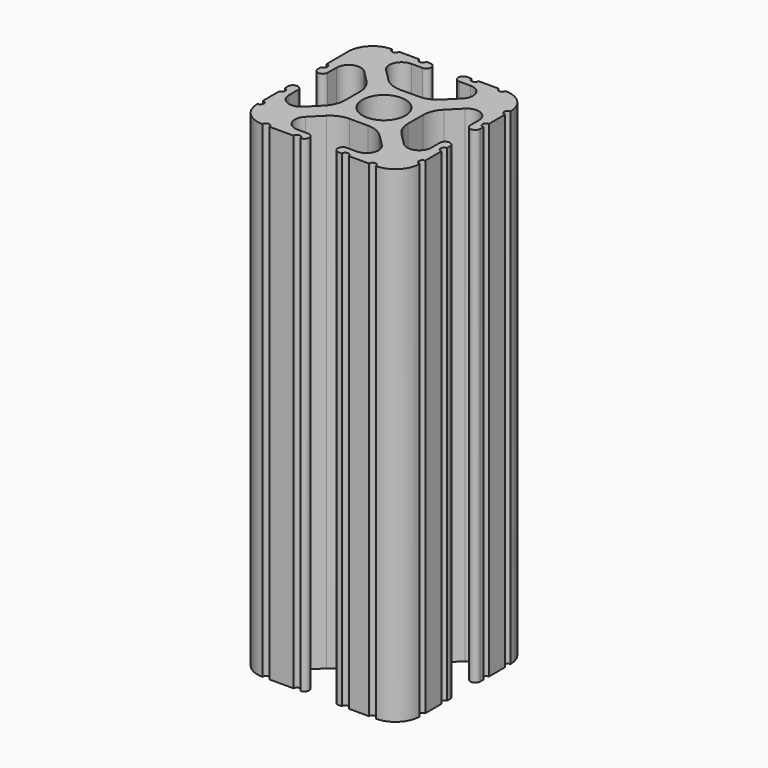
from build123d import *

# Parameters (mm, degrees)
F0_R     = 3.3625011168
F1_DEPTH = 76.2


# Not quite as in the source:
# - ends of sketch curves that miss each other by under 0.0002 mm in the source are joined


with BuildPart() as f1:
    # F0 (on Top) → F1 (new body)
    with BuildSketch(Plane.XY):
        with BuildLine():
            ThreePointArc((-8.5485764575, 18.7552378401), (-9.7846294165, 17.9293336576), (-11.2426532939, 17.6393146764))
            Line((-11.2426532939, 17.6393146764), (-14.1573467061, 17.6393146764))
            ThreePointArc((-14.1573467061, 17.6393146764), (-15.6153705835, 17.9293336576), (-16.8514235425, 18.7552378401))
            Line((-16.8514235425, 18.7552378401), (-18.696905198, 20.6007194956))
            ThreePointArc((-18.696905198, 20.6007194956), (-19.1098572893, 22.6767698525), (-17.3498667798, 23.8527579138))
            Line((-17.3498667798, 23.8527579138), (-15.6153705835, 23.8527579138))
            Line((-15.6153705835, 23.8527579138), (-15.5830195394, 23.8527579138))
            ThreePointArc((-15.5830195394, 23.8527579138), (-14.8254049311, 24.6263789569), (-15.5830195394, 25.4))
            Line((-15.5830195394, 25.4), (-15.6153705835, 25.4))
            Line((-15.6153705835, 25.4), (-16.2533409894, 25.4))
            ThreePointArc((-16.2533409894, 25.4), (-16.8016038846, 24.8587722652), (-17.3498667798, 25.4))
            Line((-17.3498667798, 25.4), (-20.4874817282, 25.4))
            ThreePointArc((-20.4874817282, 25.4), (-21.0387408641, 24.8487408595), (-21.5900000046, 25.4))
            ThreePointArc((-21.5900000046, 25.4), (-24.2840768363, 24.2840768363), (-25.4, 21.59))
            Line((-25.4, 21.59), (-25.4, 20.5047242343))
            Line((-25.4, 20.5047242343), (-25.4, 17.3498667798))
            ThreePointArc((-25.4, 17.3498667798), (-24.8441605755, 16.8026749055), (-25.4, 16.2554830313))
            Line((-25.4, 16.2554830313), (-25.4, 15.6153705835))
            ThreePointArc((-25.4, 15.6153705835), (-24.6263789569, 14.8595541131), (-23.8527579138, 15.6153705835))
            Line((-23.8527579138, 15.6153705835), (-23.8527579138, 17.3498667798))
            ThreePointArc((-23.8527579138, 17.3498667798), (-22.6767698525, 19.1098572893), (-20.6007194956, 18.696905198))
            Line((-20.6007194956, 18.696905198), (-18.7552378401, 16.8514235425))
            ThreePointArc((-18.7552378401, 16.8514235425), (-17.9293336576, 15.6153705835), (-17.6393146764, 14.1573467061))
            Line((-17.6393146764, 14.1573467061), (-17.6393146764, 11.2426532939))
            ThreePointArc((-17.6393146764, 11.2426532939), (-17.9293336576, 9.7846294165), (-18.7552378401, 8.5485764575))
            Line((-18.7552378401, 8.5485764575), (-20.6007194956, 6.703094802))
            ThreePointArc((-20.6007194956, 6.703094802), (-22.6767698525, 6.2901427107), (-23.8527579138, 8.0501332202))
            Line((-23.8527579138, 8.0501332202), (-23.8527579138, 9.7846294165))
            ThreePointArc((-23.8527579138, 9.7846294165), (-24.6263789569, 10.5582546272), (-25.4000041675, 9.7846294165))
            Line((-25.4000041675, 9.7846294165), (-25.4, 9.1492393985))
            ThreePointArc((-25.4, 9.1492393985), (-24.8993742936, 8.5996863094), (-25.4, 8.0501332202))
            Line((-25.4, 8.0501332202), (-25.4, 4.904538393))
            ThreePointArc((-25.4, 4.904538393), (-24.8462160257, 4.3572691965), (-25.4, 3.81))
            ThreePointArc((-25.4, 3.81), (-24.2840768363, 1.1159231637), (-21.59, 0))
            ThreePointArc((-21.59, 0), (-21.0408167821, 0.5548848314), (-20.4916335642, 0))
            Line((-20.4916335642, 0), (-16.7081691325, 0))
            ThreePointArc((-16.7081691325, 0), (-16.161769858, 0.5401345174), (-15.6153705835, 0))
            ThreePointArc((-15.6153705835, 0), (-14.8541835334, 0.7747), (-15.6153705835, 1.5494))
            Line((-15.6153705835, 1.5494), (-17.347708866, 1.5494))
            ThreePointArc((-17.347708866, 1.5494), (-19.1076993754, 2.7253880613), (-18.6947472842, 4.8014384182))
            Line((-18.6947472842, 4.8014384182), (-16.8514235425, 6.6447621599))
            ThreePointArc((-16.8514235425, 6.6447621599), (-15.6153705835, 7.4706663424), (-14.1573467061, 7.7606853236))
            Line((-14.1573467061, 7.7606853236), (-11.2426532939, 7.7606853236))
            ThreePointArc((-11.2426532939, 7.7606853236), (-9.7846294165, 7.4706663424), (-8.5485764575, 6.6447621599))
            Line((-8.5485764575, 6.6447621599), (-6.7052527158, 4.8014384182))
            ThreePointArc((-6.7052527158, 4.8014384182), (-6.2923006246, 2.7253880613), (-8.052291134, 1.5494))
            Line((-8.052291134, 1.5494), (-9.7846294165, 1.5494))
            ThreePointArc((-9.7846294165, 1.5494), (-10.4018355229, 0.7747), (-9.7846294165, 0))
            Line((-9.7846294165, 0), (-9.1528678313, 0))
            ThreePointArc((-9.1528678313, 0), (-8.6025794826, 0.5452621138), (-8.052291134, 0))
            Line((-8.052291134, 0), (-4.8988661729, 0))
            ThreePointArc((-4.8988661729, 0), (-4.3544330864, 0.5444330864), (-3.81, 0))
            ThreePointArc((-3.81, 0), (-1.1159231637, 1.1159231637), (0, 3.81))
            ThreePointArc((0, 3.81), (-0.5393803924, 4.3561), (0, 4.9022))
            Line((0, 4.9022), (0, 8.052291134))
            ThreePointArc((0, 8.052291134), (-0.5435172497, 8.6016602673), (0, 9.1510294005))
            Line((0, 9.1510294005), (0, 9.7846294165))
            ThreePointArc((0, 9.7846294165), (-0.7747, 10.5046907664), (-1.5494, 9.7846294165))
            Line((-1.5494, 9.7846294165), (-1.5494, 8.052291134))
            ThreePointArc((-1.5494, 8.052291134), (-2.7253880613, 6.2923006246), (-4.8014384182, 6.7052527158))
            Line((-4.8014384182, 6.7052527158), (-6.6447621599, 8.5485764575))
            ThreePointArc((-6.6447621599, 8.5485764575), (-7.4706663424, 9.7846294165), (-7.7606853236, 11.2426532939))
            Line((-7.7606853236, 11.2426532939), (-7.7606853236, 14.1573467061))
            ThreePointArc((-7.7606853236, 14.1573467061), (-7.4706663424, 15.6153705835), (-6.6447621599, 16.8514235425))
            Line((-6.6447621599, 16.8514235425), (-4.8014384182, 18.6947472842))
            ThreePointArc((-4.8014384182, 18.6947472842), (-2.7253880613, 19.1076993754), (-1.5494, 17.347708866))
            Line((-1.5494, 17.347708866), (-1.5494, 15.6153705835))
            ThreePointArc((-1.5494, 15.6153705835), (-0.7747, 14.8794054827), (0, 15.6153705835))
            Line((0, 15.6153705835), (0, 16.255508866))
            ThreePointArc((0, 16.255508866), (-0.5461, 16.801608866), (0, 17.347708866))
            Line((0, 17.347708866), (0, 20.4951651394))
            ThreePointArc((0, 20.4951651394), (-0.5510556267, 21.0425825697), (0, 21.59))
            ThreePointArc((0, 21.59), (-1.1159231637, 24.2840768363), (-3.81, 25.4))
            ThreePointArc((-3.81, 25.4), (-4.3653028659, 24.9036192847), (-4.9206057318, 25.4))
            Line((-4.9206057318, 25.4), (-8.0501332202, 25.4))
            ThreePointArc((-8.0501332202, 25.4), (-8.5963647474, 24.8594330871), (-9.1425962746, 25.4))
            Line((-9.1425962746, 25.4), (-9.7846294165, 25.4))
            Line((-9.7846294165, 25.4), (-9.856202747, 25.4))
            ThreePointArc((-9.856202747, 25.4), (-10.594864404, 24.6263789569), (-9.856202747, 23.8527579138))
            Line((-9.856202747, 23.8527579138), (-9.7846294165, 23.8527579138))
            Line((-9.7846294165, 23.8527579138), (-8.0501332202, 23.8527579138))
            ThreePointArc((-8.0501332202, 23.8527579138), (-6.2901427107, 22.6767698525), (-6.703094802, 20.6007194956))
            Line((-6.703094802, 20.6007194956), (-8.5485764575, 18.7552378401))
        make_face()
        with Locations((-12.7, 12.7)):
            Circle(F0_R, mode=Mode.SUBTRACT)
        with BuildLine():
            ThreePointArc((-9.856202747, 23.8527579138), (-9.8204160818, 23.8519306347), (-9.7846294165, 23.8527579138))
            Line((-9.7846294165, 23.8527579138), (-9.856202747, 23.8527579138))
        make_face()
        with BuildLine():
            Line((-15.5830195394, 23.8527579138), (-15.6153705835, 23.8527579138))
            ThreePointArc((-15.6153705835, 23.8527579138), (-15.5991950614, 23.8525888265), (-15.5830195394, 23.8527579138))
        make_face()
        with BuildLine():
            ThreePointArc((-9.7846294165, 25.4), (-9.8204160818, 25.4008272791), (-9.856202747, 25.4))
            Line((-9.856202747, 25.4), (-9.7846294165, 25.4))
        make_face()
        with BuildLine():
            Line((-15.6153705835, 25.4), (-15.5830195394, 25.4))
            ThreePointArc((-15.5830195394, 25.4), (-15.5991950614, 25.4001690873), (-15.6153705835, 25.4))
        make_face()
    extrude(amount=F1_DEPTH)


solid = f1.part
